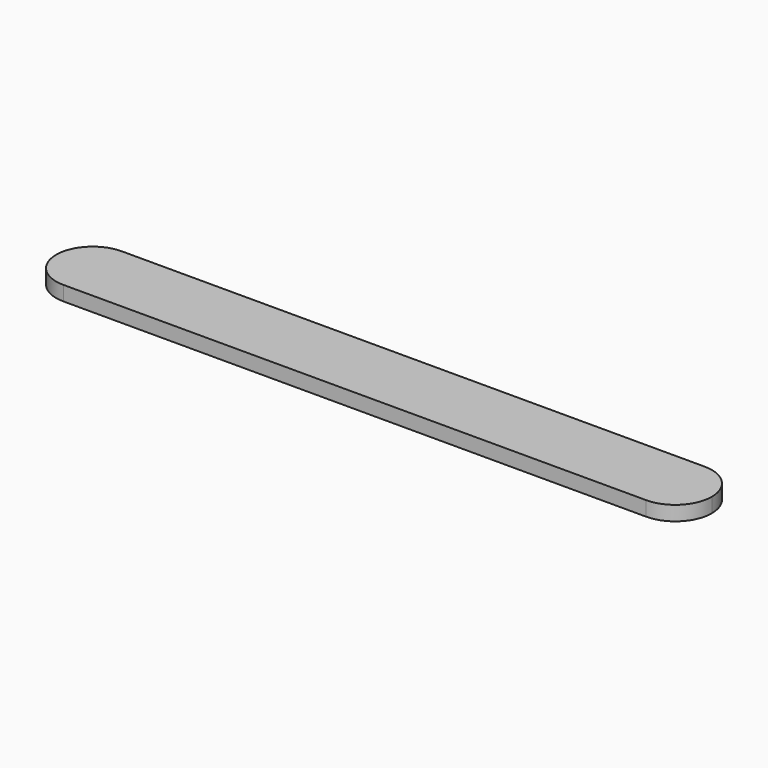
from build123d import *

# Parameters (mm, degrees)
F0_W     = 90
F0_H     = 10
F1_DEPTH = 2
F2_R     = 4.99999


# Not quite as in the source:
# - a fillet or chamfer is up to 0.001 mm smaller than in the source, because OpenCascade refuses the exact size


with BuildPart() as f1:
    # F0 (on Top) → F1 (new body)
    with BuildSketch(Plane.XY):
        with Locations((0, -5)):
            Rectangle(F0_W, F0_H)
    extrude(amount=F1_DEPTH)

    # F2 (radius 5 in the source; OpenCascade refuses exactly that, so slightly less here)
    f2_edges = [f1.edges().sort_by_distance(p)[0] for p in [
        (45, -10, 1),
        (45, 0, 1),
        (-45, 0, 1),
        (-45, -10, 1),
    ]]
    fillet(f2_edges, radius=F2_R)


solid = f1.part
